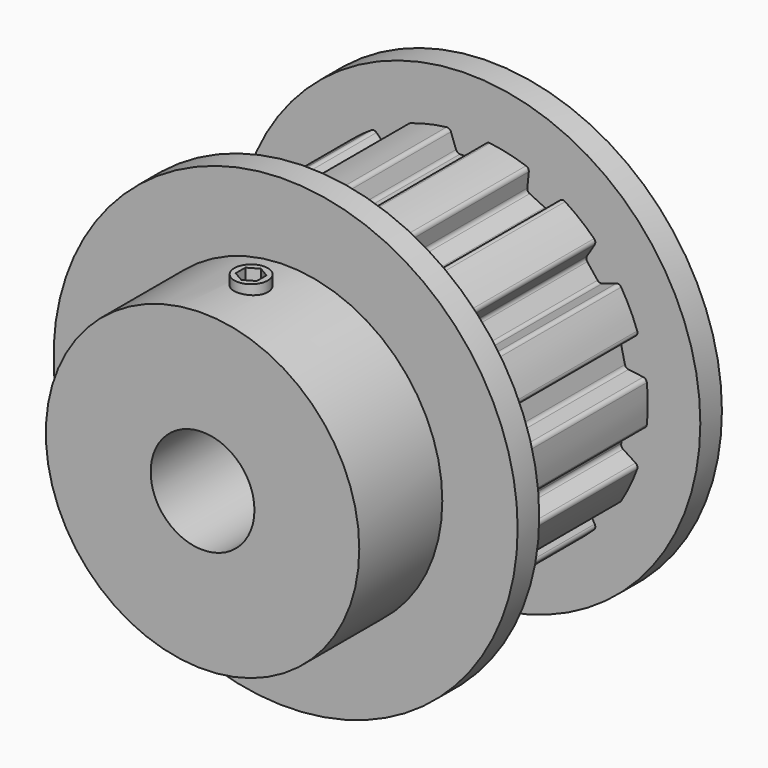
from build123d import *

# Parameters (mm, degrees)
F0_R            = 10.9855
F1_DEPTH        = 12.319
F3_DEPTH        = 25.4
F3_COPIES_COUNT = 14
F3_COPIES_ANGLE = 334.282
F4_R            = 0.254
F7_R            = 14.1986
F8_DEPTH        = 1.651
F9_R            = 14.1986
F10_DEPTH       = 1.651
F11_R           = 9.5885
F12_DEPTH       = 6.35
F13_R           = 3.175
F14_DEPTH       = 25.4
F16_R           = 1.0252013479
F17_DEPTH       = 2.54
F19_DEPTH       = 2.54


# Not quite as in the source:
# - a feature of the source that left no trace in its solid (it failed there, or was rolled back) is left out
# - a pattern or mirror of a feature is missing from the dataset's text; its kind, count and spacing are read off the source's solid


with BuildPart() as f1:
    # F0 (on Front) → F1 (new body)
    with BuildSketch(Plane.XZ):
        Circle(F0_R)
    extrude(amount=F1_DEPTH)

    # F2 (on face) → F3 (cut)
    with BuildSketch(Plane.XZ.offset(12.319)):
        with BuildLine():
            ThreePointArc((1.1269476292, 10.9275431498), (0, 10.9855), (-1.1269476292, 10.9275431498))
            Line((-1.1269476292, 10.9275431498), (-0.6858, 9.7155))
            Line((-0.6858, 9.7155), (0.6858, 9.7155))
            Line((0.6858, 9.7155), (1.1269476292, 10.9275431498))
        make_face()
    f3 = extrude(amount=-F3_DEPTH, mode=Mode.SUBTRACT)

    # F3_copies: F3 ×14 about axis
    f3_copies_axis = Axis((0, 0, 0), (0, 1, 0))
    for i in range(1, F3_COPIES_COUNT):
        add(f3.rotate(f3_copies_axis, i * F3_COPIES_ANGLE / (F3_COPIES_COUNT - 1)), mode=Mode.SUBTRACT)

    # F4
    f4_edges = [f1.edges().sort_by_distance(p)[0] for p in [
        (-1.126948, -6.1595, 10.927543),
        (1.126948, -6.1595, 10.927543),
        (-0.6858, -6.1595, 9.7155),
        (0.6858, -6.1595, 9.7155),
        (-3.726608, -6.1595, 10.334099),
        (-3.5981, -6.1595, 9.050687),
        (3.725887, -6.1595, 10.334359),
        (3.597468, -6.1595, 9.050938),
        (4.83324, -6.1595, 8.45583),
        (5.756581, -6.1595, 9.356441),
        (7.84078, -6.1595, 7.694373),
        (7.168229, -6.1595, 6.593767),
        (8.023418, -6.1595, 5.521415),
        (9.246078, -6.1595, 5.932221),
        (10.402745, -6.1595, 3.530455),
        (9.319265, -6.1595, 2.830647),
        (9.624495, -6.1595, 1.493441),
        (10.904316, -6.1595, 1.333078),
        (10.904363, -6.1595, -1.332697),
        (9.624547, -6.1595, -1.493105),
        (9.319364, -6.1595, -2.830322),
        (10.402868, -6.1595, -3.530092),
        (9.246286, -6.1595, -5.931898),
        (8.023611, -6.1595, -5.521135),
        (7.168459, -6.1595, -6.593516),
        (7.841049, -6.1595, -7.694099),
        (5.756908, -6.1595, -9.35624),
        (4.833535, -6.1595, -8.455661),
        (3.597784, -6.1595, -9.050813),
        (3.726248, -6.1595, -10.334229),
        (1.127329, -6.1595, -10.927504),
        (0.686139, -6.1595, -9.715476),
        (-0.685461, -6.1595, -9.715524),
        (-1.126566, -6.1595, -10.927582),
        (-3.725526, -6.1595, -10.334489),
        (-3.597152, -6.1595, -9.051064),
        (-4.832945, -6.1595, -8.455998),
        (-5.756255, -6.1595, -9.356642),
        (-7.840512, -6.1595, -7.694647),
        (-7.167999, -6.1595, -6.594017),
        (-8.023225, -6.1595, -5.521695),
        (-9.245871, -6.1595, -5.932544),
        (-10.402621, -6.1595, -3.530819),
        (-9.319166, -6.1595, -2.830972),
        (-9.624443, -6.1595, -1.493777),
        (-10.90427, -6.1595, -1.333458),
        (-10.904409, -6.1595, 1.332316),
        (-9.624599, -6.1595, 1.492769),
        (-9.319463, -6.1595, 2.829996),
        (-10.402991, -6.1595, 3.529729),
        (-9.246493, -6.1595, 5.931575),
        (-8.023803, -6.1595, 5.520855),
        (-7.168689, -6.1595, 6.593266),
        (-7.841317, -6.1595, 7.693826),
        (-5.757235, -6.1595, 9.356039),
        (-4.83383, -6.1595, 8.455492),
    ]]
    fillet(f4_edges, radius=F4_R)

    # F7 (on face) → F8 (join)
    with BuildSketch(Plane.XZ.offset(12.319)):
        Circle(F7_R)
        with BuildLine():
            Line((-1.0585699305, 10.7396769666), (-0.746629211, 9.8826268836))
            ThreePointArc((-0.746629211, 9.8826268836), (-0.6536357001, 9.7614353808), (-0.5079472853, 9.7155))
            Line((-0.5079472853, 9.7155), (0.5079472853, 9.7155))
            ThreePointArc((0.5079472853, 9.7155), (0.6536357001, 9.7614353808), (0.746629211, 9.8826268836))
            Line((0.746629211, 9.8826268836), (1.0585699305, 10.7396769666))
            ThreePointArc((1.0585699305, 10.7396769666), (1.1644295938, 10.8693084613), (1.3279560421, 10.9049412195))
            ThreePointArc((1.3279560421, 10.9049412195), (2.4444770163, 10.7100766742), (3.5349777521, 10.4012087058))
            ThreePointArc((3.5349777521, 10.4012087058), (3.6668500306, 10.2981538908), (3.7059821055, 10.1354293584))
            Line((3.7059821055, 10.1354293584), (3.6151754133, 9.2279074568))
            ThreePointArc((3.6151754133, 9.2279074568), (3.6463773947, 9.078369469), (3.7577080278, 8.973771842))
            Line((3.7577080278, 8.973771842), (4.6729996069, 8.5329962714))
            ThreePointArc((4.6729996069, 8.5329962714), (4.8241910567, 8.5111715392), (4.960557994, 8.5800136181))
            Line((4.960557994, 8.5800136181), (5.6134637899, 9.2168463112))
            ThreePointArc((5.6134637899, 9.2168463112), (5.7650846952, 9.2877102218), (5.9278776022, 9.2488635725))
            ThreePointArc((5.9278776022, 9.2488635725), (6.849282974, 8.5888609834), (7.6977811455, 7.837434254))
            ThreePointArc((7.6977811455, 7.837434254), (7.7718809029, 7.6873682062), (7.7365349713, 7.5237795212))
            Line((7.7365349713, 7.5237795212), (7.2609658534, 6.7455277166))
            ThreePointArc((7.2609658534, 6.7455277166), (7.2241965054, 6.5972604293), (7.2791194411, 6.4547169463))
            Line((7.2791194411, 6.4547169463), (7.912527267, 5.6604649052))
            ThreePointArc((7.912527267, 5.6604649052), (8.0392770851, 5.5752026215), (8.1920088946, 5.5780605563))
            Line((8.1920088946, 5.5780605563), (9.0565665919, 5.8685460902))
            ThreePointArc((9.0565665919, 5.8685460902), (9.2239190154, 5.8666072566), (9.3537359539, 5.7609750872))
            ThreePointArc((9.3537359539, 5.7609750872), (9.8975340762, 4.7665532054), (10.3359778861, 3.7213937428))
            ThreePointArc((10.3359778861, 3.7213937428), (10.3376290772, 3.554038234), (10.2348056814, 3.4219854339))
            Line((10.2348056814, 3.4219854339), (9.4686643763, 2.9271426731))
            ThreePointArc((9.4686643763, 2.9271426731), (9.37120616, 2.8095115994), (9.3588434751, 2.6572541285))
            Line((9.3588434751, 2.6572541285), (9.5849161004, 1.6668335377))
            ThreePointArc((9.5849161004, 1.6668335377), (9.6621204793, 1.5350205744), (9.8009674139, 1.4713283285))
            Line((9.8009674139, 1.4713283285), (10.7059444987, 1.3579337375))
            ThreePointArc((10.7059444987, 1.3579337375), (10.8558829648, 1.2835761613), (10.9270126597, 1.1320797612))
            ThreePointArc((10.9270126597, 1.1320797612), (10.9854999983, 0.0001917331), (10.92705217, -1.1316983358))
            ThreePointArc((10.92705217, -1.1316983358), (10.8559277634, -1.2831972187), (10.7059918931, -1.3575600287))
            Line((10.7059918931, -1.3575600287), (9.801018767, -1.4709862093))
            ThreePointArc((9.801018767, -1.4709862093), (9.6621740558, -1.5346833018), (9.5849742781, -1.66649896))
            Line((9.5849742781, -1.66649896), (9.3589362251, -2.6569274416))
            ThreePointArc((9.3589362251, -2.6569274416), (9.3713042248, -2.8091844808), (9.468766547, -2.9268121526))
            Line((9.468766547, -2.9268121526), (10.234925125, -3.4216281697))
            ThreePointArc((10.234925125, -3.4216281697), (10.3377531302, -3.5536773805), (10.3361077809, -3.7210329468))
            ThreePointArc((10.3361077809, -3.7210329468), (9.8977004543, -4.7662077134), (9.3539370442, -5.7606485767))
            ThreePointArc((9.3539370442, -5.7606485767), (9.224123793, -5.8662852775), (9.0567714373, -5.8682299528))
            Line((9.0567714373, -5.8682299528), (8.1922036006, -5.5777745979))
            ThreePointArc((8.1922036006, -5.5777745979), (8.0394716915, -5.5749219944), (7.9127248497, -5.6601887025))
            Line((7.9127248497, -5.6601887025), (7.2793447488, -6.4544628531))
            ThreePointArc((7.2793447488, -6.4544628531), (7.2244267889, -6.5970082533), (7.2612013123, -6.7452742569))
            Line((7.2612013123, -6.7452742569), (7.736797596, -7.5235094606))
            ThreePointArc((7.736797596, -7.5235094606), (7.7721492379, -7.6870969117), (7.6980547189, -7.837165546))
            ThreePointArc((7.6980547189, -7.837165546), (6.8495827776, -8.5886218931), (5.9282004449, -9.2486566449))
            ThreePointArc((5.9282004449, -9.2486566449), (5.7654088939, -9.2875089767), (5.6137855151, -9.2166503588))
            Line((5.6137855151, -9.2166503588), (4.96085749, -8.5798404568))
            ThreePointArc((4.96085749, -8.5798404568), (4.8244881497, -8.511003138), (4.6732974618, -8.5328331478))
            Line((4.6732974618, -8.5328331478), (3.7580212692, -8.9736406678))
            ThreePointArc((3.7580212692, -8.9736406678), (3.6466942874, -9.0782421809), (3.6154975258, -9.2277812577))
            Line((3.6154975258, -9.2277812577), (3.7063358965, -10.1352999891))
            ThreePointArc((3.7063358965, -10.1352999891), (3.6672095018, -10.2980258874), (3.5353408206, -10.4010853055))
            ThreePointArc((3.5353408206, -10.4010853055), (2.444850867, -10.7099913393), (1.3283366956, -10.9048948584))
            ThreePointArc((1.3283366956, -10.9048948584), (1.1648090036, -10.8692678085), (1.0589448153, -10.739640009))
            Line((1.0589448153, -10.739640009), (0.7469741793, -9.8826008153))
            ThreePointArc((0.7469741793, -9.8826008153), (0.6539764381, -9.7614125586), (0.5082864199, -9.7154822634))
            Line((0.5082864199, -9.7154822634), (-0.5076081501, -9.7155177248))
            ThreePointArc((-0.5076081501, -9.7155177248), (-0.6532949614, -9.761458191), (-0.7462842418, -9.8826529399))
            Line((-0.7462842418, -9.8826529399), (-1.0581950444, -10.7397139112))
            ThreePointArc((-1.0581950444, -10.7397139112), (-1.1640501827, -10.869349101), (-1.327575387, -10.9049875672))
            ThreePointArc((-1.327575387, -10.9049875672), (-2.4441031626, -10.710161996), (-3.5346146793, -10.4013320935))
            ThreePointArc((-3.5346146793, -10.4013320935), (-3.666490555, -10.2982818818), (-3.70562831, -10.1355587154))
            Line((-3.70562831, -10.1355587154), (-3.6148532963, -9.2280336446))
            ThreePointArc((-3.6148532963, -9.2280336446), (-3.6460604976, -9.0784967461), (-3.7573947817, -8.9739030053))
            Line((-3.7573947817, -8.9739030053), (-4.6727017463, -8.5331593847))
            ThreePointArc((-4.6727017463, -8.5331593847), (-4.8238939578, -8.51133993), (-4.960258492, -8.580186769))
            Line((-4.960258492, -8.580186769), (-5.6131420579, -9.2170422525))
            ThreePointArc((-5.6131420579, -9.2170422525), (-5.7647604894, -9.2879114556), (-5.9275547524, -9.2490704888))
            ThreePointArc((-5.9275547524, -9.2490704888), (-6.848983162, -8.5891000633), (-7.6975075627, -7.8377029525))
            ThreePointArc((-7.6975075627, -7.8377029525), (-7.7716125584, -7.6876394914), (-7.7362723371, -7.5240495727))
            Line((-7.7362723371, -7.5240495727), (-7.2607303856, -6.745781168))
            ThreePointArc((-7.2607303856, -6.745781168), (-7.2239662132, -6.5975125973), (-7.2788941246, -6.4549710315))
            Line((-7.2788941246, -6.4549710315), (-7.9123296747, -5.6607411011))
            ThreePointArc((-7.9123296747, -5.6607411011), (-8.0390824689, -5.5754832418), (-8.1918141785, -5.578346508))
            Line((-8.1918141785, -5.578346508), (-9.0563617355, -5.8688622204))
            ThreePointArc((-9.0563617355, -5.8688622204), (-9.2237142266, -5.8669292286), (-9.3535348522, -5.7613015906))
            ThreePointArc((-9.3535348522, -5.7613015906), (-9.8973676861, -4.7668986916), (-10.3358479786, -3.7217545342))
            ThreePointArc((-10.3358479786, -3.7217545342), (-10.3375050116, -3.5543990832), (-10.2346862253, -3.422342694))
            Line((-10.2346862253, -3.422342694), (-9.4685621939, -2.9274731901))
            ThreePointArc((-9.4685621939, -2.9274731901), (-9.3711080839, -2.8098387145), (-9.3587507137, -2.6575808121))
            Line((-9.3587507137, -2.6575808121), (-9.5848579111, -1.6671681134))
            ThreePointArc((-9.5848579111, -1.6671681134), (-9.6620668911, -1.5353578451), (-9.8009160489, -1.471670446))
            Line((-9.8009160489, -1.471670446), (-10.7058970914, -1.3583074446))
            ThreePointArc((-10.7058970914, -1.3583074446), (-10.8558381529, -1.2839551023), (-10.926973136, -1.1324611852))
            ThreePointArc((-10.926973136, -1.1324611852), (-10.9854999849, -0.0005751994), (-10.9270916671, 1.131316909))
            ThreePointArc((-10.9270916671, 1.131316909), (-10.8559725488, 1.2828182745), (-10.7060392743, 1.3571863183))
            Line((-10.7060392743, 1.3571863183), (-9.8010701081, 1.4706440884))
            ThreePointArc((-9.8010701081, 1.4706440884), (-9.6622276204, 1.5343460274), (-9.585032444, 1.6661643803))
            Line((-9.585032444, 1.6661643803), (-9.3590289636, 2.6566007515))
            ThreePointArc((-9.3590289636, 2.6566007515), (-9.3714022781, 2.8088573589), (-9.4688687063, 2.9264816285))
            Line((-9.4688687063, 2.9264816285), (-10.2350445561, 3.4212709014))
            ThreePointArc((-10.2350445561, 3.4212709014), (-10.3378771707, 3.5533165227), (-10.3362376632, 3.7206721463))
            ThreePointArc((-10.3362376632, 3.7206721463), (-9.8978668203, 4.7658622156), (-9.354138123, 5.7603220592))
            ThreePointArc((-9.354138123, 5.7603220592), (-9.2243285594, 5.8659632913), (-9.0569762716, 5.8679138082))
            Line((-9.0569762716, 5.8679138082), (-8.1923982967, 5.5774886326))
            ThreePointArc((-8.1923982967, 5.5774886326), (-8.0396662881, 5.5746413605), (-7.9129224227, 5.6599124928))
            Line((-7.9129224227, 5.6599124928), (-7.2795700476, 6.4542087521))
            ThreePointArc((-7.2795700476, 6.4542087521), (-7.2246570635, 6.5967560692), (-7.2614367624, 6.7450207891))
            Line((-7.2614367624, 6.7450207891), (-7.7370602113, 7.5232393909))
            ThreePointArc((-7.7370602113, 7.5232393909), (-7.7724175635, 7.6868256079), (-7.6983282829, 7.8368968284))
            ThreePointArc((-7.6983282829, 7.8368968284), (-6.8498825729, 8.5883827923), (-5.9285232803, 9.2484497061))
            ThreePointArc((-5.9285232803, 9.2484497061), (-5.7657330856, 9.2873077203), (-5.6141072335, 9.2164543951))
            Line((-5.6141072335, 9.2164543951), (-4.9611569799, 8.5796672849))
            ThreePointArc((-4.9611569799, 8.5796672849), (-4.8247852368, 8.5108347264), (-4.6735953111, 8.5326700137))
            Line((-4.6735953111, 8.5326700137), (-3.7583345061, 8.9735094827))
            ThreePointArc((-3.7583345061, 8.9735094827), (-3.6470111756, 9.0781148817), (-3.6158196339, 9.2276550474))
            Line((-3.6158196339, 9.2276550474), (-3.7066896829, 10.1351706074))
            ThreePointArc((-3.7066896829, 10.1351706074), (-3.6675689685, 10.2978978713), (-3.5357038848, 10.4009618925))
            ThreePointArc((-3.5357038848, 10.4009618925), (-2.444850867, 10.7099913393), (-1.3279560421, 10.9049412195))
            ThreePointArc((-1.3279560421, 10.9049412195), (-1.1644295938, 10.8693084613), (-1.0585699305, 10.7396769666))
        make_face(mode=Mode.SUBTRACT)
        with BuildLine():
            ThreePointArc((-0.5079472853, 9.7155), (-0.6536357001, 9.7614353808), (-0.746629211, 9.8826268836))
            Line((-0.746629211, 9.8826268836), (-1.0585699305, 10.7396769666))
            ThreePointArc((-1.0585699305, 10.7396769666), (-1.1644295938, 10.8693084613), (-1.3279560421, 10.9049412195))
            ThreePointArc((-1.3279560421, 10.9049412195), (-2.444850867, 10.7099913393), (-3.5357038848, 10.4009618925))
            ThreePointArc((-3.5357038848, 10.4009618925), (-3.6675689685, 10.2978978713), (-3.7066896829, 10.1351706074))
            Line((-3.7066896829, 10.1351706074), (-3.6158196339, 9.2276550474))
            ThreePointArc((-3.6158196339, 9.2276550474), (-3.6470111756, 9.0781148817), (-3.7583345061, 8.9735094827))
            Line((-3.7583345061, 8.9735094827), (-4.6735953111, 8.5326700137))
            ThreePointArc((-4.6735953111, 8.5326700137), (-4.8247852368, 8.5108347264), (-4.9611569799, 8.5796672849))
            Line((-4.9611569799, 8.5796672849), (-5.6141072335, 9.2164543951))
            ThreePointArc((-5.6141072335, 9.2164543951), (-5.7657330856, 9.2873077203), (-5.9285232803, 9.2484497061))
            ThreePointArc((-5.9285232803, 9.2484497061), (-6.8498825729, 8.5883827923), (-7.6983282829, 7.8368968284))
            ThreePointArc((-7.6983282829, 7.8368968284), (-7.7724175635, 7.6868256079), (-7.7370602113, 7.5232393909))
            Line((-7.7370602113, 7.5232393909), (-7.2614367624, 6.7450207891))
            ThreePointArc((-7.2614367624, 6.7450207891), (-7.2246570635, 6.5967560692), (-7.2795700476, 6.4542087521))
            Line((-7.2795700476, 6.4542087521), (-7.9129224227, 5.6599124928))
            ThreePointArc((-7.9129224227, 5.6599124928), (-8.0396662881, 5.5746413605), (-8.1923982967, 5.5774886326))
            Line((-8.1923982967, 5.5774886326), (-9.0569762716, 5.8679138082))
            ThreePointArc((-9.0569762716, 5.8679138082), (-9.2243285594, 5.8659632913), (-9.354138123, 5.7603220592))
            ThreePointArc((-9.354138123, 5.7603220592), (-9.8978668203, 4.7658622156), (-10.3362376632, 3.7206721463))
            ThreePointArc((-10.3362376632, 3.7206721463), (-10.3378771707, 3.5533165227), (-10.2350445561, 3.4212709014))
            Line((-10.2350445561, 3.4212709014), (-9.4688687063, 2.9264816285))
            ThreePointArc((-9.4688687063, 2.9264816285), (-9.3714022781, 2.8088573589), (-9.3590289636, 2.6566007515))
            Line((-9.3590289636, 2.6566007515), (-9.585032444, 1.6661643803))
            ThreePointArc((-9.585032444, 1.6661643803), (-9.6622276204, 1.5343460274), (-9.8010701081, 1.4706440884))
            Line((-9.8010701081, 1.4706440884), (-10.7060392743, 1.3571863183))
            ThreePointArc((-10.7060392743, 1.3571863183), (-10.8559725488, 1.2828182745), (-10.9270916671, 1.131316909))
            ThreePointArc((-10.9270916671, 1.131316909), (-10.9854999849, -0.0005751994), (-10.926973136, -1.1324611852))
            ThreePointArc((-10.926973136, -1.1324611852), (-10.8558381529, -1.2839551023), (-10.7058970914, -1.3583074446))
            Line((-10.7058970914, -1.3583074446), (-9.8009160489, -1.471670446))
            ThreePointArc((-9.8009160489, -1.471670446), (-9.6620668911, -1.5353578451), (-9.5848579111, -1.6671681134))
            Line((-9.5848579111, -1.6671681134), (-9.3587507137, -2.6575808121))
            ThreePointArc((-9.3587507137, -2.6575808121), (-9.3711080839, -2.8098387145), (-9.4685621939, -2.9274731901))
            Line((-9.4685621939, -2.9274731901), (-10.2346862253, -3.422342694))
            ThreePointArc((-10.2346862253, -3.422342694), (-10.3375050116, -3.5543990832), (-10.3358479786, -3.7217545342))
            ThreePointArc((-10.3358479786, -3.7217545342), (-9.8973676861, -4.7668986916), (-9.3535348522, -5.7613015906))
            ThreePointArc((-9.3535348522, -5.7613015906), (-9.2237142266, -5.8669292286), (-9.0563617355, -5.8688622204))
            Line((-9.0563617355, -5.8688622204), (-8.1918141785, -5.578346508))
            ThreePointArc((-8.1918141785, -5.578346508), (-8.0390824689, -5.5754832418), (-7.9123296747, -5.6607411011))
            Line((-7.9123296747, -5.6607411011), (-7.2788941246, -6.4549710315))
            ThreePointArc((-7.2788941246, -6.4549710315), (-7.2239662132, -6.5975125973), (-7.2607303856, -6.745781168))
            Line((-7.2607303856, -6.745781168), (-7.7362723371, -7.5240495727))
            ThreePointArc((-7.7362723371, -7.5240495727), (-7.7716125584, -7.6876394914), (-7.6975075627, -7.8377029525))
            ThreePointArc((-7.6975075627, -7.8377029525), (-6.848983162, -8.5891000633), (-5.9275547524, -9.2490704888))
            ThreePointArc((-5.9275547524, -9.2490704888), (-5.7647604894, -9.2879114556), (-5.6131420579, -9.2170422525))
            Line((-5.6131420579, -9.2170422525), (-4.960258492, -8.580186769))
            ThreePointArc((-4.960258492, -8.580186769), (-4.8238939578, -8.51133993), (-4.6727017463, -8.5331593847))
            Line((-4.6727017463, -8.5331593847), (-3.7573947817, -8.9739030053))
            ThreePointArc((-3.7573947817, -8.9739030053), (-3.6460604976, -9.0784967461), (-3.6148532963, -9.2280336446))
            Line((-3.6148532963, -9.2280336446), (-3.70562831, -10.1355587154))
            ThreePointArc((-3.70562831, -10.1355587154), (-3.666490555, -10.2982818818), (-3.5346146793, -10.4013320935))
            ThreePointArc((-3.5346146793, -10.4013320935), (-2.4441031626, -10.710161996), (-1.327575387, -10.9049875672))
            ThreePointArc((-1.327575387, -10.9049875672), (-1.1640501827, -10.869349101), (-1.0581950444, -10.7397139112))
            Line((-1.0581950444, -10.7397139112), (-0.7462842418, -9.8826529399))
            ThreePointArc((-0.7462842418, -9.8826529399), (-0.6532949614, -9.761458191), (-0.5076081501, -9.7155177248))
            Line((-0.5076081501, -9.7155177248), (0.5082864199, -9.7154822634))
            ThreePointArc((0.5082864199, -9.7154822634), (0.6539764381, -9.7614125586), (0.7469741793, -9.8826008153))
            Line((0.7469741793, -9.8826008153), (1.0589448153, -10.739640009))
            ThreePointArc((1.0589448153, -10.739640009), (1.1648090036, -10.8692678085), (1.3283366956, -10.9048948584))
            ThreePointArc((1.3283366956, -10.9048948584), (2.444850867, -10.7099913393), (3.5353408206, -10.4010853055))
            ThreePointArc((3.5353408206, -10.4010853055), (3.6672095018, -10.2980258874), (3.7063358965, -10.1352999891))
            Line((3.7063358965, -10.1352999891), (3.6154975258, -9.2277812577))
            ThreePointArc((3.6154975258, -9.2277812577), (3.6466942874, -9.0782421809), (3.7580212692, -8.9736406678))
            Line((3.7580212692, -8.9736406678), (4.6732974618, -8.5328331478))
            ThreePointArc((4.6732974618, -8.5328331478), (4.8244881497, -8.511003138), (4.96085749, -8.5798404568))
            Line((4.96085749, -8.5798404568), (5.6137855151, -9.2166503588))
            ThreePointArc((5.6137855151, -9.2166503588), (5.7654088939, -9.2875089767), (5.9282004449, -9.2486566449))
            ThreePointArc((5.9282004449, -9.2486566449), (6.8495827776, -8.5886218931), (7.6980547189, -7.837165546))
            ThreePointArc((7.6980547189, -7.837165546), (7.7721492379, -7.6870969117), (7.736797596, -7.5235094606))
            Line((7.736797596, -7.5235094606), (7.2612013123, -6.7452742569))
            ThreePointArc((7.2612013123, -6.7452742569), (7.2244267889, -6.5970082533), (7.2793447488, -6.4544628531))
            Line((7.2793447488, -6.4544628531), (7.9127248497, -5.6601887025))
            ThreePointArc((7.9127248497, -5.6601887025), (8.0394716915, -5.5749219944), (8.1922036006, -5.5777745979))
            Line((8.1922036006, -5.5777745979), (9.0567714373, -5.8682299528))
            ThreePointArc((9.0567714373, -5.8682299528), (9.224123793, -5.8662852775), (9.3539370442, -5.7606485767))
            ThreePointArc((9.3539370442, -5.7606485767), (9.8977004543, -4.7662077134), (10.3361077809, -3.7210329468))
            ThreePointArc((10.3361077809, -3.7210329468), (10.3377531302, -3.5536773805), (10.234925125, -3.4216281697))
            Line((10.234925125, -3.4216281697), (9.468766547, -2.9268121526))
            ThreePointArc((9.468766547, -2.9268121526), (9.3713042248, -2.8091844808), (9.3589362251, -2.6569274416))
            Line((9.3589362251, -2.6569274416), (9.5849742781, -1.66649896))
            ThreePointArc((9.5849742781, -1.66649896), (9.6621740558, -1.5346833018), (9.801018767, -1.4709862093))
            Line((9.801018767, -1.4709862093), (10.7059918931, -1.3575600287))
            ThreePointArc((10.7059918931, -1.3575600287), (10.8559277634, -1.2831972187), (10.92705217, -1.1316983358))
            ThreePointArc((10.92705217, -1.1316983358), (10.9854999983, 0.0001917331), (10.9270126597, 1.1320797612))
            ThreePointArc((10.9270126597, 1.1320797612), (10.8558829648, 1.2835761613), (10.7059444987, 1.3579337375))
            Line((10.7059444987, 1.3579337375), (9.8009674139, 1.4713283285))
            ThreePointArc((9.8009674139, 1.4713283285), (9.6621204793, 1.5350205744), (9.5849161004, 1.6668335377))
            Line((9.5849161004, 1.6668335377), (9.3588434751, 2.6572541285))
            ThreePointArc((9.3588434751, 2.6572541285), (9.37120616, 2.8095115994), (9.4686643763, 2.9271426731))
            Line((9.4686643763, 2.9271426731), (10.2348056814, 3.4219854339))
            ThreePointArc((10.2348056814, 3.4219854339), (10.3376290772, 3.554038234), (10.3359778861, 3.7213937428))
            ThreePointArc((10.3359778861, 3.7213937428), (9.8975340762, 4.7665532054), (9.3537359539, 5.7609750872))
            ThreePointArc((9.3537359539, 5.7609750872), (9.2239190154, 5.8666072566), (9.0565665919, 5.8685460902))
            Line((9.0565665919, 5.8685460902), (8.1920088946, 5.5780605563))
            ThreePointArc((8.1920088946, 5.5780605563), (8.0392770851, 5.5752026215), (7.912527267, 5.6604649052))
            Line((7.912527267, 5.6604649052), (7.2791194411, 6.4547169463))
            ThreePointArc((7.2791194411, 6.4547169463), (7.2241965054, 6.5972604293), (7.2609658534, 6.7455277166))
            Line((7.2609658534, 6.7455277166), (7.7365349713, 7.5237795212))
            ThreePointArc((7.7365349713, 7.5237795212), (7.7718809029, 7.6873682062), (7.6977811455, 7.837434254))
            ThreePointArc((7.6977811455, 7.837434254), (6.849282974, 8.5888609834), (5.9278776022, 9.2488635725))
            ThreePointArc((5.9278776022, 9.2488635725), (5.7650846952, 9.2877102218), (5.6134637899, 9.2168463112))
            Line((5.6134637899, 9.2168463112), (4.960557994, 8.5800136181))
            ThreePointArc((4.960557994, 8.5800136181), (4.8241910567, 8.5111715392), (4.6729996069, 8.5329962714))
            Line((4.6729996069, 8.5329962714), (3.7577080278, 8.973771842))
            ThreePointArc((3.7577080278, 8.973771842), (3.6463773947, 9.078369469), (3.6151754133, 9.2279074568))
            Line((3.6151754133, 9.2279074568), (3.7059821055, 10.1354293584))
            ThreePointArc((3.7059821055, 10.1354293584), (3.6668500306, 10.2981538908), (3.5349777521, 10.4012087058))
            ThreePointArc((3.5349777521, 10.4012087058), (2.4444770163, 10.7100766742), (1.3279560421, 10.9049412195))
            ThreePointArc((1.3279560421, 10.9049412195), (1.1644295938, 10.8693084613), (1.0585699305, 10.7396769666))
            Line((1.0585699305, 10.7396769666), (0.746629211, 9.8826268836))
            ThreePointArc((0.746629211, 9.8826268836), (0.6536357001, 9.7614353808), (0.5079472853, 9.7155))
            Line((0.5079472853, 9.7155), (-0.5079472853, 9.7155))
        make_face()
    extrude(amount=F8_DEPTH)

    # F9 (on Front) → F10 (join)
    with BuildSketch(Plane.XZ):
        Circle(F9_R)
    extrude(amount=-F10_DEPTH)

    # F11 (on face) → F12 (join)
    with BuildSketch(Plane.XZ.offset(13.97)):
        Circle(F11_R)
    extrude(amount=F12_DEPTH)

    # F13 (on face) → F14 (cut)
    with BuildSketch(Plane.XZ.offset(20.32)):
        Circle(F13_R)
    extrude(amount=-F14_DEPTH, mode=Mode.SUBTRACT)

    # F16 (on offset) → F17 (join)
    with BuildSketch(Plane.XY.offset(10.16)):
        with Locations((0, -16.6069511324)):
            Circle(F16_R)
    extrude(amount=-F17_DEPTH)

    # F18 (on face) → F19 (cut)
    with BuildSketch(Plane.XY.offset(10.16)):
        Polygon((0.6453618024, -16.2343513221), (0, -15.8617515117), (-0.6453618024, -16.2343513221), (-0.6453618024, -16.9795509428), (0, -17.3521507531), (0.6453618024, -16.9795509428), align=None)
    extrude(amount=-F19_DEPTH, mode=Mode.SUBTRACT)


solid = f1.part
